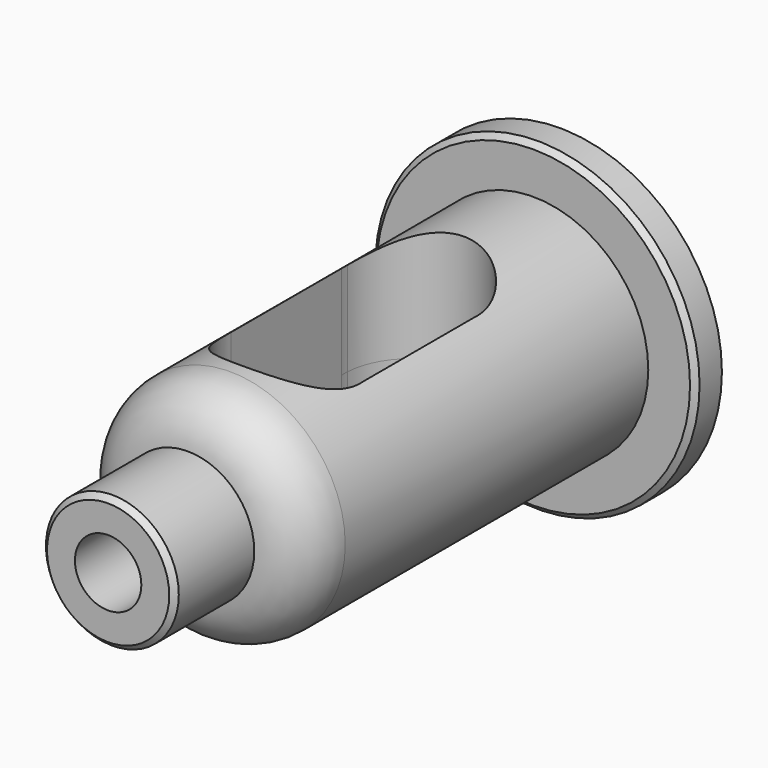
from build123d import *

# Parameters (mm, degrees)
F0_R          = 11
F1_DEPTH      = 44.45
F0_R_2        = 15.5
F2_DEPTH      = 3.175
F3_R          = 6.35
F4_DEPTH      = 9.525
F7_DEPTH      = 25.4
F7_DEPTH_BACK = 25.4
F8_R          = 3.175
F9_DEPTH      = 25.4
F10_SIZE      = 0.508


# Not quite as in the source:
# - a fillet or chamfer that OpenCascade refuses, or shapes differently, is made with other operations: its cross-section is extruded or revolved along the edge and cut away or added


with BuildPart() as f1:
    # F0 (on Front) → F1 (new body)
    with BuildSketch(Plane.XZ):
        Circle(F0_R)
    extrude(amount=F1_DEPTH)

    # F0 (on Front) → F2 (join)
    with BuildSketch(Plane.XZ):
        Circle(F0_R_2)
        Circle(F0_R, mode=Mode.SUBTRACT)
    extrude(amount=F2_DEPTH)

    # F3 (on face) → F4 (join)
    with BuildSketch(Plane.XZ.offset(44.45)):
        Circle(F3_R)
    extrude(amount=F4_DEPTH)

    # F5: fillet of radius 5.08 on 1 edges, made by hand

    # F5_s1 → F5_t2 (revolve, cut)
    with BuildSketch(Plane.XY):
        with BuildLine():
            ThreePointArc((11, -39.3882315343), (9.6610426354, -42.8249450807), (6.35, -44.45))
            Line((6.35, -44.45), (11, -44.45))
            Line((11, -44.45), (11, -39.3882315343))
        make_face()
    revolve(axis=Axis((0, -44.45, 0), (0, -1, 0)), mode=Mode.SUBTRACT)

    # F6 (on Top) → F7 (cut, two sides)
    with BuildSketch(Plane.XY) as f7_sk:
        with BuildLine():
            Line((-6.3399745388, -32.1066831191), (-6.3399745388, -31.3933168809))
            ThreePointArc((-6.3399745388, -31.3933168809), (-6.35, -31.75), (-6.3399745388, -32.1066831191))
        make_face()
        with BuildLine():
            Line((-6.3399745388, -18.1366831191), (-6.3399745388, -31.3933168809))
            Line((-6.3399745388, -31.3933168809), (-6.3399745388, -32.1066831191))
            ThreePointArc((-6.3399745388, -32.1066831191), (0, -38.1), (6.3399745388, -32.1066831191))
            Line((6.3399745388, -32.1066831191), (6.3399745388, -31.3933168809))
            Line((6.3399745388, -31.3933168809), (6.3399745388, -18.1366831191))
            Line((6.3399745388, -18.1366831191), (6.3399745388, -17.4233168809))
            ThreePointArc((6.3399745388, -17.4233168809), (0, -11.43), (-6.3399745388, -17.4233168809))
            Line((-6.3399745388, -17.4233168809), (-6.3399745388, -18.1366831191))
        make_face()
        with BuildLine():
            ThreePointArc((-6.3399745388, -17.4233168809), (-6.35, -17.78), (-6.3399745388, -18.1366831191))
            Line((-6.3399745388, -18.1366831191), (-6.3399745388, -17.4233168809))
        make_face()
        with BuildLine():
            Line((6.3399745388, -31.3933168809), (6.3399745388, -32.1066831191))
            ThreePointArc((6.3399745388, -32.1066831191), (6.35, -31.75), (6.3399745388, -31.3933168809))
        make_face()
        with BuildLine():
            ThreePointArc((6.3399745388, -18.1366831191), (6.35, -17.78), (6.3399745388, -17.4233168809))
            Line((6.3399745388, -17.4233168809), (6.3399745388, -18.1366831191))
        make_face()
    extrude(amount=-F7_DEPTH, mode=Mode.SUBTRACT)
    extrude(f7_sk.sketch, amount=F7_DEPTH_BACK, mode=Mode.SUBTRACT)

    # F8 (on face) → F9 (cut)
    with BuildSketch(Plane.XZ.offset(53.975)):
        Circle(F8_R)
    extrude(amount=-F9_DEPTH, mode=Mode.SUBTRACT)

    # F10
    f10_edges = [f1.edges().sort_by_distance(p)[0] for p in [
        (-15.5, -3.175, 0),
        (-6.35, -53.975, 0),
    ]]
    chamfer(f10_edges, length=F10_SIZE)


solid = f1.part
